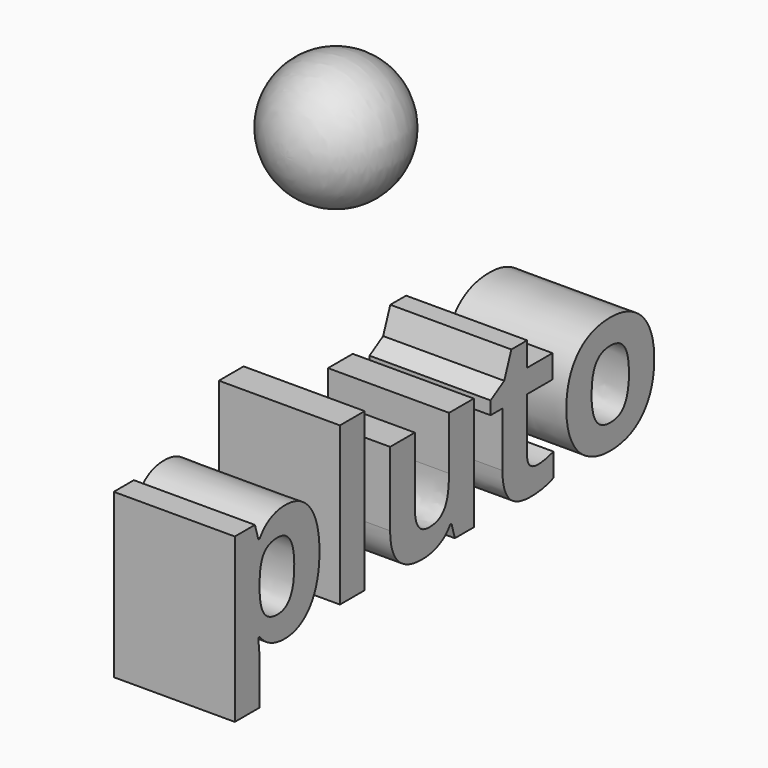
from build123d import *

# Parameters (mm, degrees)
F2_TEXT_SIZE = 87.1123952998
F3_DEPTH     = 50.8


# Not quite as in the source:
# - Text() gives the source's letters only with a copy of the font that has no kerning and outlines rounded to 1/6400 em; it was checked with that copy


with BuildPart() as f1:
    # F0 (on Top) → F1 (revolve)
    with BuildSketch(Plane.XY):
        with BuildLine():
            Line((0, 53.3164963126), (0, 0))
            ThreePointArc((0, 0), (26.7637505424, 26.6582481563), (0, 53.3164963126))
        make_face()
    revolve(axis=Axis((0, 26.6582481563, 0), (0, 1, 0)))


with BuildPart() as f3:
    # F2 (on Right) → F3 (new body)
    with BuildSketch(Plane.YZ):
        with Locations((-96.6789796948, -134.7045302391)):
            Text('pluto', F2_TEXT_SIZE, font='Open Sans', font_style=FontStyle.BOLD, text_align=(TextAlign.LEFT, TextAlign.BOTTOM))
    extrude(amount=F3_DEPTH)


solid = Compound([f1.part, f3.part])
